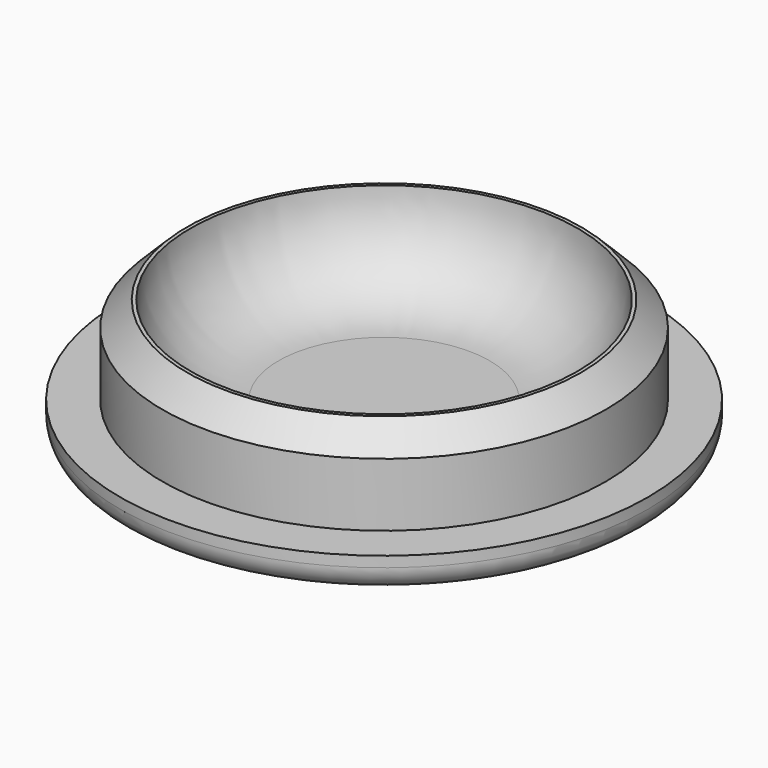
from build123d import *

# Parameters (mm, degrees)
F0_R     = 15
F0_R_2   = 13
F0_R_3   = 12.6
F0_R_4   = 11
F1_DEPTH = 2
F2_DEPTH = 7
F3_R     = 4.99999
F4_SIZE  = 1.4
F5_R     = 1.4


# Not quite as in the source:
# - a fillet or chamfer is up to 0.001 mm smaller than in the source, because OpenCascade refuses the exact size


with BuildPart() as f1:
    # F0 (on Top) → F1 (new body)
    with BuildSketch(Plane.XY):
        Circle(F0_R)
        Circle(F0_R_2, mode=Mode.SUBTRACT)
        Circle(F0_R_2)
        Circle(F0_R_3, mode=Mode.SUBTRACT)
        Circle(F0_R_3)
        Circle(F0_R_4, mode=Mode.SUBTRACT)
        Circle(F0_R_4)
    extrude(amount=F1_DEPTH)

    # F0 (on Top) → F2 (join)
    with BuildSketch(Plane.XY):
        Circle(F0_R_3)
        Circle(F0_R_4, mode=Mode.SUBTRACT)
    extrude(amount=F2_DEPTH)

    # F3 (radius 5 in the source; OpenCascade refuses exactly that, so slightly less here)
    f3_edges = [f1.edges().sort_by_distance(p)[0] for p in [
        (-11, 0, 2),
    ]]
    fillet(f3_edges, radius=F3_R)

    # F4
    f4_edges = [f1.edges().sort_by_distance(p)[0] for p in [
        (-12.6, 0, 7),
    ]]
    chamfer(f4_edges, length=F4_SIZE)

    # F5
    f5_edges = [f1.edges().sort_by_distance(p)[0] for p in [
        (-15, 0, 0),
    ]]
    fillet(f5_edges, radius=F5_R)


solid = f1.part
